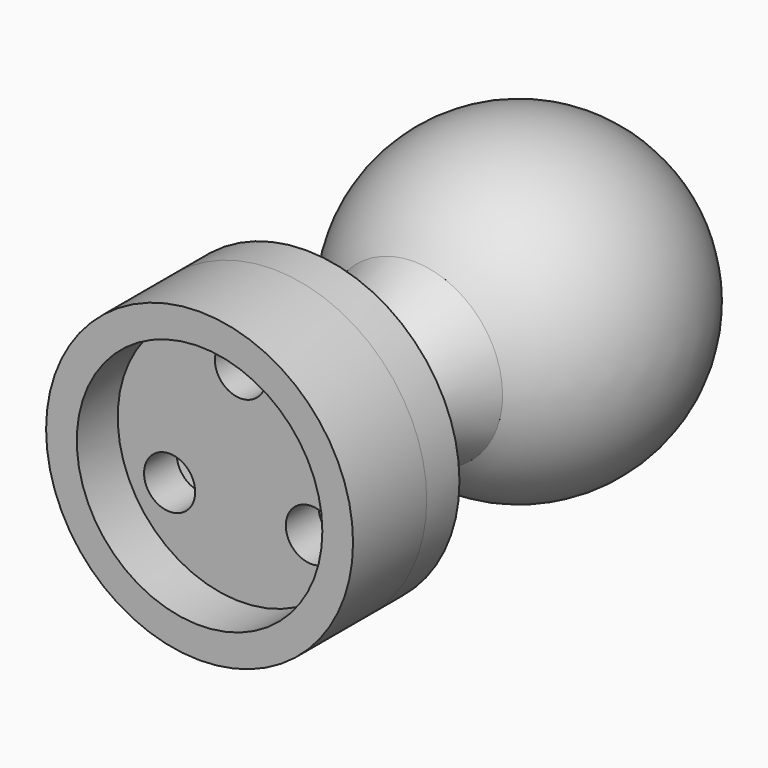
from build123d import *

# Parameters (mm, degrees)
F0_R         = 9.525
F0_R_2       = 1.5875
F1_DEPTH     = 2.54
F2_R         = 9.525
F2_R_2       = 7.62
F3_DEPTH     = 3.175
F4_R         = 9.525
F4_R_2       = 7.747
F5_DEPTH     = 2.54
F6_R         = 3.175
F7_DEPTH     = 12.7
F10_R        = 2.54
F11_DEPTH    = 27.9544081902
F12_T2_ANGLE = 180
F12_T4_ANGLE = 180


# Not quite as in the source:
# - a fillet or chamfer that OpenCascade refuses, or shapes differently, is made with other operations: its cross-section is extruded or revolved along the edge and cut away or added


with BuildPart() as f1:
    # F0 (on Front) → F1 (new body)
    with BuildSketch(Plane.XZ):
        Circle(F0_R)
        with Locations((-4.3994090512, -2.54)):
            Circle(F0_R_2, mode=Mode.SUBTRACT)
        with Locations((4.3994090512, -2.54)):
            Circle(F0_R_2, mode=Mode.SUBTRACT)
        with Locations((0, 5.08)):
            Circle(F0_R_2, mode=Mode.SUBTRACT)
    extrude(amount=F1_DEPTH)

    # F2 (on face) → F3 (join)
    with BuildSketch(Plane.XZ.offset(2.54)):
        Circle(F2_R)
        Circle(F2_R_2, mode=Mode.SUBTRACT)
    extrude(amount=F3_DEPTH)

    # F4 (on face) → F5 (join)
    with BuildSketch(Plane(origin=(0, 0, 0), x_dir=(-1, 0, 0), z_dir=(0, 1, 0))):
        Circle(F4_R)
        Circle(F4_R_2, mode=Mode.SUBTRACT)
    extrude(amount=F5_DEPTH)

    # F6 (on face) → F7 (join)
    with BuildSketch(Plane(origin=(0, 0, 0), x_dir=(-1, 0, 0), z_dir=(0, 1, 0))):
        Circle(F6_R)
    extrude(amount=F7_DEPTH)

    # F8 (on Top) → F9 (revolve)
    with BuildSketch(Plane.XY):
        with BuildLine():
            Line((0, 27.9505403934), (0, 9.2075))
            ThreePointArc((0, 9.2075), (9.6048581812, 16.9002312755), (4.1957274517, 27.9534081902))
            Line((4.1957274517, 27.9534081902), (0, 27.9505403934))
        make_face()
    revolve(axis=Axis((0, 12.9395495169, 0), (0, -1, 0)))

    # F10 (on face) → F11 (cut, through all)
    with BuildSketch(Plane(origin=(0, 0, 0), x_dir=(-1, 0, 0), z_dir=(0, 1, 0))):
        Circle(F10_R)
    extrude(amount=F11_DEPTH, mode=Mode.SUBTRACT)

    # F12: chamfer of 3.81 on 2 edges, made by hand

    # F12_s1 → F12_t2 (revolve)
    with BuildSketch(Plane.XY):
        with BuildLine():
            Line((-3.1035480311, 6.3541505323), (-5.586882311, 11.0326284828))
            Line((-5.586882311, 11.0326284828), (-5.5441822052, 11.0957406129))
            ThreePointArc((-5.5441822052, 11.0957406129), (-4.405806786, 10.3339526014), (-3.1504193548, 9.8057870222))
            Line((-3.1504193548, 9.8057870222), (-3.0988, 9.733660523))
            ThreePointArc((-3.0988, 9.733660523), (-3.0988, 8.0439055277), (-3.0273480311, 6.3541505323))
            Line((-3.0273480311, 6.3541505323), (-3.1035480311, 6.3541505323))
        make_face()
    revolve(axis=Axis((0, 9.733660523, 0), (0, -1, 0)), revolution_arc=F12_T2_ANGLE)

    # F12_s3 → F12_t4 (revolve)
    with BuildSketch(Plane.XY):
        with BuildLine():
            Line((3.1035480311, 6.3541505323), (5.586882311, 11.0326284828))
            Line((5.586882311, 11.0326284828), (5.5441822052, 11.0957406129))
            ThreePointArc((5.5441822052, 11.0957406129), (4.405806786, 10.3339526014), (3.1504193548, 9.8057870222))
            Line((3.1504193548, 9.8057870222), (3.0988, 9.733660523))
            ThreePointArc((3.0988, 9.733660523), (3.0988, 8.0439055277), (3.0273480311, 6.3541505323))
            Line((3.0273480311, 6.3541505323), (3.1035480311, 6.3541505323))
        make_face()
    revolve(axis=Axis((0, 9.733660523, 0), (0, -1, 0)), revolution_arc=F12_T4_ANGLE)


solid = f1.part
